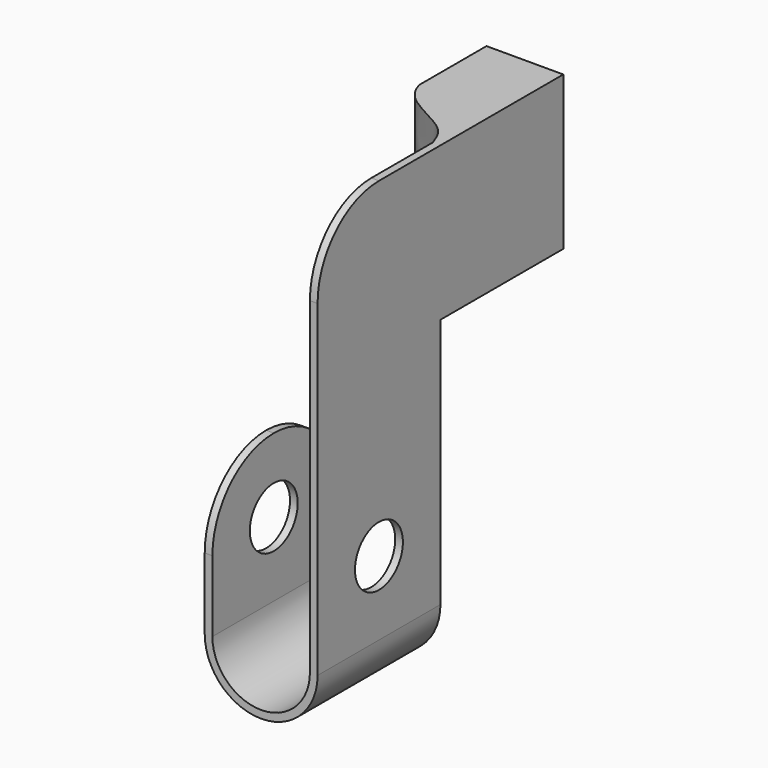
from build123d import *

# Parameters (mm, degrees)
F1_DEPTH  = 10
F0_W      = 0.5
F0_H      = 10
F2_DEPTH  = 10
F3_DEPTH  = 10
F4_R      = 1.95
F5_DEPTH  = 25
F6_DEPTH  = 25
F7_R      = 4.99999
F4_W      = 10
F4_H      = 10
F8_DEPTH  = 4.5
F10_DEPTH = 25


# Not quite as in the source:
# - a fillet or chamfer is up to 0.001 mm smaller than in the source, because OpenCascade refuses the exact size


with BuildPart() as f1:
    # F0 (on Front) → F1 (new body)
    with BuildSketch(Plane.XZ):
        with BuildLine():
            Line((0.5, 3.675), (0, 3.675))
            ThreePointArc((0, 3.675), (3.675, 0), (7.35, 3.675))
            Line((7.35, 3.675), (7.35, 20))
            Line((7.35, 20), (6.85, 20))
            Line((6.85, 20), (6.85, 3.675))
            ThreePointArc((6.85, 3.675), (3.675, 0.5), (0.5, 3.675))
        make_face()
        Polygon((0, 11.5236516859), (0, 3.675), (0.5, 3.675), (0.5, 13.3078707406), (0, 13.3078707406), align=None)
    extrude(amount=F1_DEPTH)

    # F0 (on Front) → F2 (join)
    with BuildSketch(Plane.XZ):
        with Locations((7.1, 25)):
            Rectangle(F0_W, F0_H)
    extrude(amount=F2_DEPTH)

    # F0 (on Front) → F3 (join)
    with BuildSketch(Plane.XZ):
        with Locations((7.1, 25)):
            Rectangle(F0_W, F0_H)
    extrude(amount=-F3_DEPTH)

    # F4 (on face) → F5 (cut)
    with BuildSketch(Plane(origin=(6.85, 0, 0), x_dir=(0, -1, 0), z_dir=(-1, 0, 0))):
        with Locations((5.0057064388, 8.4952701442)):
            Circle(F4_R)
    extrude(amount=-F5_DEPTH, mode=Mode.SUBTRACT)

    # F4 (on face) → F6 (cut)
    with BuildSketch(Plane(origin=(6.85, 0, 0), x_dir=(0, -1, 0), z_dir=(-1, 0, 0))):
        with Locations((5.0057064388, 8.4952701442)):
            Circle(F4_R)
    extrude(amount=F6_DEPTH, mode=Mode.SUBTRACT)

    # F7 (radius 5 in the source; OpenCascade refuses exactly that, so slightly less here)
    f7_edges = [f1.edges().sort_by_distance(p)[0] for p in [
        (7.1, -10, 30),
        (0.25, -10, 13.307871),
        (0.25, 0, 13.307871),
    ]]
    fillet(f7_edges, radius=F7_R)

    # F4 (on face) → F8 (join)
    with BuildSketch(Plane(origin=(6.85, 0, 0), x_dir=(0, -1, 0), z_dir=(-1, 0, 0))):
        with Locations((-5, 25)):
            Rectangle(F4_W, F4_H)
    extrude(amount=F8_DEPTH)

    # F9 (on face) → F10 (cut)
    with BuildSketch(Plane.XY.offset(30)):
        with BuildLine():
            Line((2.35, 0), (6.85, 0))
            add(Edge.make_bspline(
                [(6.85, 0), (6.6607907806, 0.4988620131), (6.3387521568, 1.6560182736), (2.9528697619, 2.8701009159), (2.4258734683, 4.2211432066), (2.35, 4.5559741557)],
                knots=[0, 0, 0, 0, 0.2515030108, 0.6187434404, 0.8676489933, 0.8676489933, 0.8676489933, 0.8676489933], degree=3))
            Line((2.35, 4.5559741557), (2.35, 0))
        make_face()
    extrude(amount=-F10_DEPTH, mode=Mode.SUBTRACT)


solid = f1.part
